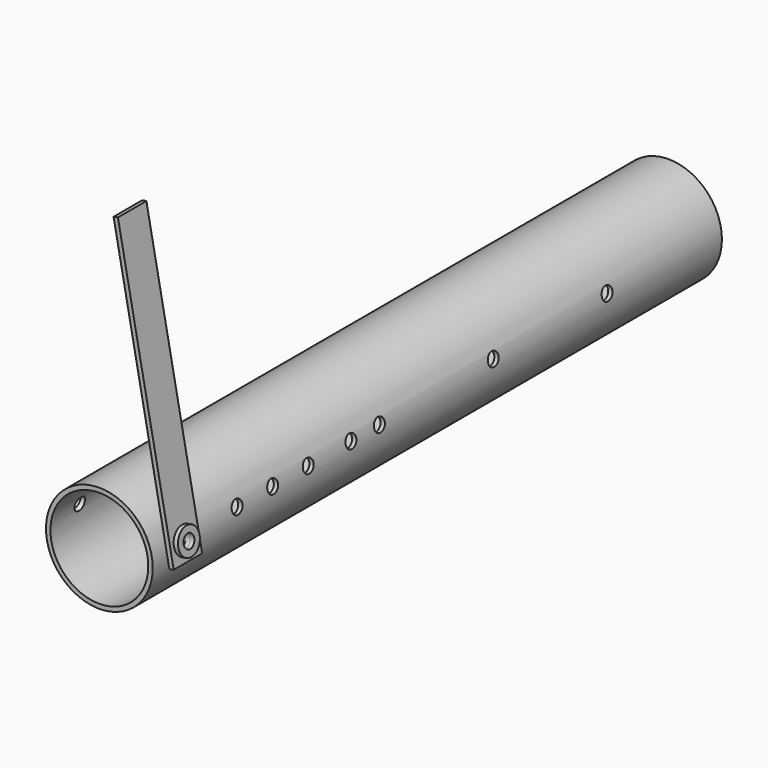
from build123d import *

# Parameters (mm, degrees)
F0_R          = 38.1
F0_R_2        = 34.925
F1_DEPTH      = 508
F4_DEPTH      = 12.7
F5_R          = 4.7625
F6_DEPTH      = 38.1
F6_DEPTH_BACK = 42.2755644605
F7_R          = 9.525
F7_R_2        = 4.7625
F8_DEPTH      = 3.175


# Not quite as in the source:
# - a pattern or mirror of a feature is missing from the dataset's text; its kind, count and spacing are read off the source's solid


with BuildPart() as f1:
    # F0 (on Front) → F1 (new body)
    with BuildSketch(Plane.XZ):
        Circle(F0_R)
        Circle(F0_R_2, mode=Mode.SUBTRACT)
    extrude(amount=-F1_DEPTH)


with BuildPart() as f4:
    # F3 (on offset) → F4 (new body, symmetric)
    with BuildSketch(Plane.XZ.offset(-25.4)):
        Polygon((3.118690114, 203.7953125), (0, 203.2), (39.8055313684, -5.3310104561), (42.9242214824, -4.7356979561), align=None)
    extrude(amount=F4_DEPTH, both=True)


with BuildPart() as f6_tool:
    # F5 (on face) → F6 (new body, two sides)
    with BuildSketch(Plane(origin=(37.4242813684, 0, 7.14375), x_dir=(0, -1, 0), z_dir=(-0.9822646028, 0, -0.1875))) as f6_sk:
        with Locations((-25.4, 0)):
            Circle(F5_R)
        with Locations((-139.7, 0)):
            Circle(F5_R)
        with Locations((-177.8, 0)):
            Circle(F5_R)
        with Locations((-304.8, 0)):
            Circle(F5_R)
        with Locations((-406.4, 0)):
            Circle(F5_R)
        with Locations((-76.2, 0)):
            Circle(F5_R)
        with Locations((-203.2, 0)):
            Circle(F5_R)
        with Locations((-107.95, 0)):
            Circle(F5_R)
    f6 = extrude(amount=F6_DEPTH) + extrude(f6_sk.sketch, amount=-F6_DEPTH_BACK)


with BuildPart() as f1_1:
    add(f1.part)

    # F6: cut by f6_tool
    add(f6_tool.part, mode=Mode.SUBTRACT)

    # F6_copies: F6 across plane
    add(f6.mirror(Plane(origin=(-1e-05, 0, 0), x_dir=(-5e-06, 0, -1), z_dir=(-1, 0, 5e-06))), mode=Mode.SUBTRACT)


with BuildPart() as f4_1:
    add(f4.part)

    # F6: cut by f6_tool
    add(f6_tool.part, mode=Mode.SUBTRACT)


with BuildPart() as f8:
    # F7 (on face) → F8 (new body)
    with BuildSketch(Plane(origin=(40.5429714824, 0, 7.7390625), x_dir=(0, 1, 0), z_dir=(0.9822646028, 0, 0.1875))):
        with Locations((25.4, 0)):
            Circle(F7_R)
        with Locations((25.4, 0)):
            Circle(F7_R_2, mode=Mode.SUBTRACT)
    extrude(amount=F8_DEPTH)


solid = Compound([f1_1.part, f4_1.part, f8.part])
